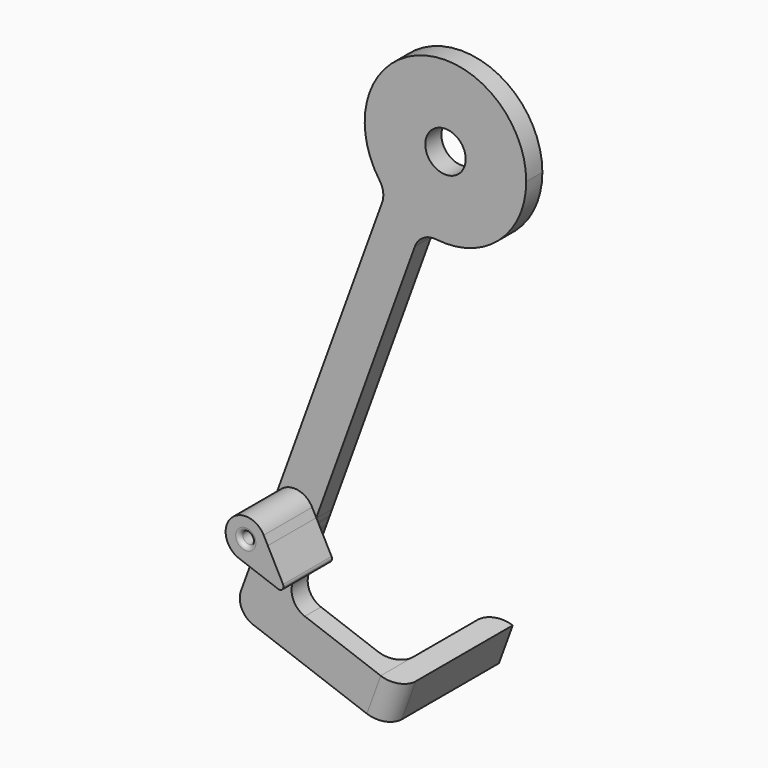
from build123d import *

# Parameters (mm, degrees)
F0_R     = 5
F0_R_2   = 1.5
F1_DEPTH = 5
F2_DEPTH = 30
F4_R     = 4.99999
F5_R     = 5
F3_R     = 1.5
F6_DEPTH = 15
F7_R     = 1
F7_2_R   = 1


# Not quite as in the source:
# - a fillet or chamfer is up to 0.001 mm smaller than in the source, because OpenCascade refuses the exact size
# - a feature names something its author has since deleted; it is built from what else it names


with BuildPart() as f1:
    # F0 (on Front) → F1 (new body)
    with BuildSketch(Plane.XZ):
        with BuildLine():
            ThreePointArc((20, 33.8170940264), (-7.2600924867, 52.4528407806), (-14.7291057085, 20.287369527))
            ThreePointArc((-14.7291057085, 20.287369527), (-10.7719287617, 16.9658166044), (-6.0959419995, 14.7687478741))
            ThreePointArc((-6.0959419995, 14.7687478741), (11.7915469725, 17.6628555734), (20, 33.8170940264))
        make_face()
        with Locations((0, 33.8170940264)):
            Circle(F0_R, mode=Mode.SUBTRACT)
        with BuildLine():
            Line((-14.7291057085, 20.287369527), (-42.1496687283, -55.0500081989))
            ThreePointArc((-42.1496687283, -55.0500081989), (-36.7371185286, -51.8113638601), (-32.4609528428, -56.4480570615))
            Line((-32.4609528428, -56.4480570615), (-32.0687023036, -56.5908245822))
            Line((-32.0687023036, -56.5908245822), (-6.0959419995, 14.7687478741))
            ThreePointArc((-6.0959419995, 14.7687478741), (-10.7719287617, 16.9658166044), (-14.7291057085, 20.287369527))
        make_face()
        with BuildLine():
            ThreePointArc((-32.4512056942, -56.7601091071), (-32.5271669199, -57.628349943), (-32.7527425538, -58.4702097236))
            Line((-32.7527425538, -58.4702097236), (-32.5817325186, -58.0003635134))
            Line((-32.5817325186, -58.0003635134), (-32.0687023036, -56.5908245822))
            Line((-32.0687023036, -56.5908245822), (-32.4609528428, -56.4480570615))
            ThreePointArc((-32.4609528428, -56.4480570615), (-32.4536430754, -56.6040069883), (-32.4512056942, -56.7601091071))
        make_face()
        with BuildLine():
            ThreePointArc((-33.8290334161, -60.2068275447), (-33.2012405407, -59.3940787717), (-32.7527425538, -58.4702097236))
            ThreePointArc((-32.7527425538, -58.4702097236), (-32.5271669199, -57.628349943), (-32.4512056942, -56.7601091071))
            ThreePointArc((-32.4512056942, -56.7601091071), (-32.4536430754, -56.6040069883), (-32.4609528428, -56.4480570615))
            ThreePointArc((-32.4609528428, -56.4480570615), (-36.7371185286, -51.8113638601), (-42.1496687283, -55.0500081989))
            ThreePointArc((-42.1496687283, -55.0500081989), (-40.0851754907, -61.0100741788), (-33.8290334161, -60.2068275447))
        make_face()
        with Locations((-37.4512056942, -56.7601091071)):
            Circle(F0_R_2, mode=Mode.SUBTRACT)
        with BuildLine():
            Line((-39.5341938332, -77.1020939848), (-33.6077929485, -60.8194413757))
            Line((-33.6077929485, -60.8194413757), (-33.4367828769, -60.3495950653))
            Line((-33.4367828769, -60.3495950653), (-33.8290334161, -60.2068275447))
            ThreePointArc((-33.8290334161, -60.2068275447), (-40.0851754907, -61.0100741788), (-42.1496687283, -55.0500081989))
            Line((-42.1496687283, -55.0500081989), (-42.3206788698, -55.5198547009))
            Line((-42.3206788698, -55.5198547009), (-52.3513214743, -83.0788187594))
            Line((-52.3513214743, -83.0788187594), (-42.9543952664, -86.4990201927))
            Line((-42.9543952664, -86.4990201927), (-39.5341938332, -77.1020939848))
        make_face()
        with BuildLine():
            Line((-33.8290334161, -60.2068275447), (-33.4367828769, -60.3495950653))
            Line((-33.4367828769, -60.3495950653), (-32.7527425538, -58.4702097236))
            ThreePointArc((-32.7527425538, -58.4702097236), (-33.2012405407, -59.3940787717), (-33.8290334161, -60.2068275447))
        make_face()
        Polygon((-16.0418783135, -85.652597568), (-39.5341938332, -77.1020939848), (-42.9543952664, -86.4990201927), (-19.4620797468, -95.0495237758), align=None)
        Polygon((-11.3434152096, -87.3626982846), (-16.0418783135, -85.652597568), (-19.4620797468, -95.0495237758), (-14.7636166428, -96.7596244924), align=None)
    extrude(amount=F1_DEPTH)

    # F0 (on Front) → F2 (join)
    with BuildSketch(Plane.XZ):
        Polygon((-11.3434152096, -87.3626982846), (-16.0418783135, -85.652597568), (-19.4620797468, -95.0495237758), (-14.7636166428, -96.7596244924), align=None)
    extrude(amount=-F2_DEPTH)

    # F4 (radius 5 in the source; OpenCascade refuses exactly that, so slightly less here)
    f4_edges = [f1.edges().sort_by_distance(p)[0] for p in [
        (-52.351321, -2.5, -83.078819),
        (-13.053516, -5, -92.061161),
        (-17.751979, 30, -90.351061),
        (-17.751979, 0, -90.351061),
        (-39.534194, -2.5, -77.102094),
    ]]
    fillet(f4_edges, radius=F4_R)

    # F5
    f5_edges = [f1.edges().sort_by_distance(p)[0] for p in [
        (-6.095942, -2.5, 14.768748),
        (-14.729106, -2.5, 20.28737),
    ]]
    fillet(f5_edges, radius=F5_R)

    # F7
    f7_edges = [f1.edges().sort_by_distance(p)[0] for p in [
        (-38.951206, -5, -56.760109),
    ]]
    fillet(f7_edges, radius=F7_R)


with BuildPart() as f6:
    # F3 (on face) → F6 (new body)
    with BuildSketch(Plane.XZ.offset(5)):
        with BuildLine():
            ThreePointArc((-32.7527426235, -58.470209915), (-32.5271669375, -57.6283500433), (-32.4512056942, -56.7601091071))
            ThreePointArc((-32.4512056942, -56.7601091071), (-32.5962642376, -55.5644739399), (-33.0230230754, -54.438213611))
            ThreePointArc((-33.0230230754, -54.438213611), (-37.7856244233, -51.7713052311), (-42.149668581, -55.050007794))
            ThreePointArc((-42.149668581, -55.050007794), (-41.9827447635, -58.8732001282), (-39.1613064108, -61.458572211))
            ThreePointArc((-39.1613064108, -61.458572211), (-35.3381144295, -61.2916480628), (-32.7527426235, -58.470209915))
        make_face()
        with Locations((-37.4512056942, -56.7601091071)):
            Circle(F3_R, mode=Mode.SUBTRACT)
        with BuildLine():
            ThreePointArc((-33.0230230754, -54.438213611), (-32.5962642376, -55.5644739399), (-32.4512056942, -56.7601091071))
            ThreePointArc((-32.4512056942, -56.7601091071), (-32.5271669375, -57.6283500433), (-32.7527426235, -58.470209915))
            Line((-32.7527426235, -58.470209915), (-31.9972492992, -56.3945090662))
            Line((-31.9972492992, -56.3945090662), (-33.0230230754, -54.438213611))
        make_face()
        with BuildLine():
            Line((-34.4628433069, -63.1686729277), (-32.7527426235, -58.470209915))
            ThreePointArc((-32.7527426235, -58.470209915), (-35.3381144295, -61.2916480628), (-39.1613064108, -61.458572211))
            Line((-39.1613064108, -61.458572211), (-34.4628433069, -63.1686729277))
        make_face()
        Polygon((-31.9972492992, -56.3945090662), (-32.7527426235, -58.470209915), (-34.4628433069, -63.1686729277), (-27.0259488145, -65.8754811583), align=None)
    extrude(amount=F6_DEPTH)

    # F7#2
    f7_2_edges = [f6.edges().sort_by_distance(p)[0] for p in [
        (-27.025949, -12.5, -65.875481),
        (-38.951206, -20, -56.760109),
    ]]
    fillet(f7_2_edges, radius=F7_2_R)


solid = Compound([f1.part, f6.part])
